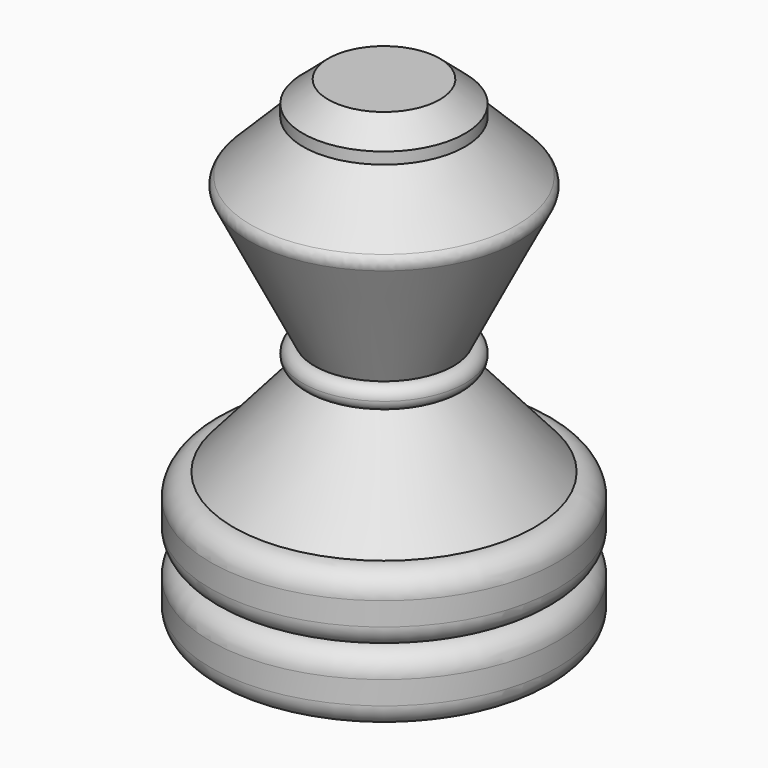
from build123d import *

# Parameters (mm, degrees)
F2_R = 2.49999
F3_R = 4.99999
F0_W = 37.5
F0_H = 15
F5_R = 4.9999


# Not quite as in the source:
# - a fillet or chamfer is up to 0.001 mm smaller than in the source, because OpenCascade refuses the exact size


with BuildPart() as f1:
    # F0 (on Front) → F1 (revolve)
    with BuildSketch(Plane.XZ):
        Polygon((0, 104.6807143092), (0, 55), (15, 55), (30, 85), (17.5, 97.5), (17.5, 100), (12.0391666392, 104.6807143092), align=None)
        Polygon((0, 55), (0, 50), (15, 50), (17.5, 50), (17.5, 55), (15, 55), align=None)
        Polygon((0, 50), (0, 30), (32.5, 30), (15, 50), align=None)
        Polygon((0, 30), (0, 15), (37.5, 15), (37.5, 30), (32.5, 30), align=None)
    revolve(axis=Axis((0, 0, 79.8403571546), (0, 0, 1)))

    # F2 (radius 2.5 in the source; OpenCascade refuses exactly that, so slightly less here)
    f2_edges = [f1.edges().sort_by_distance(p)[0] for p in [
        (-30, 0, 85),
        (-17.5, 0, 55),
        (-17.5, 0, 50),
    ]]
    fillet(f2_edges, radius=F2_R)

    # F3 (radius 5 in the source; OpenCascade refuses exactly that, so slightly less here)
    f3_edges = [f1.edges().sort_by_distance(p)[0] for p in [
        (-37.5, 0, 30),
        (-37.5, 0, 15),
    ]]
    fillet(f3_edges, radius=F3_R)

    # F0 (on Front) → F4 (revolve)
    with BuildSketch(Plane.XZ):
        with Locations((18.75, 7.5)):
            Rectangle(F0_W, F0_H)
    revolve(axis=Axis((0, 0, 7.5), (0, 0, 1)))

    # F5 (radius 5 in the source; OpenCascade refuses exactly that, so slightly less here)
    f5_edges = [f1.edges().sort_by_distance(p)[0] for p in [
        (-37.5, 0, 15),
        (-37.5, 0, 0),
    ]]
    fillet(f5_edges, radius=F5_R)


solid = f1.part
